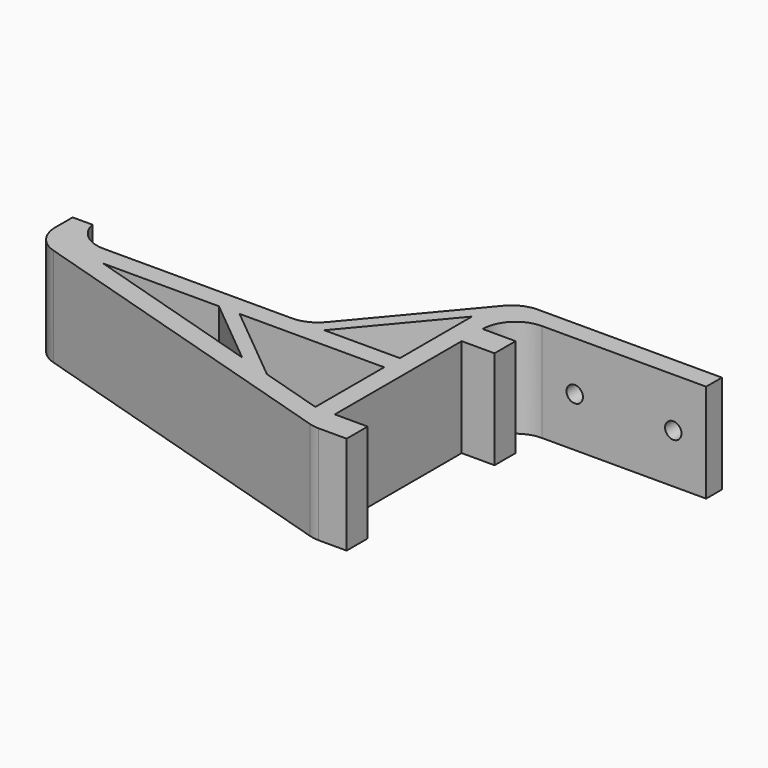
from build123d import *

# Parameters (mm, degrees)
F1_DEPTH    = 15
F2_R        = 1.25
F3_DEPTH    = 40.1383324758
F4_R        = 5
F5_W        = 4
F5_H        = 15
F6_DEPTH    = 5
F8_DEPTH    = 15
F9_T1_DEPTH = 15
F9_T3_DEPTH = 15
F9_T5_DEPTH = 33.4938424429
F9_T7_DEPTH = 18.7397003757


# Not quite as in the source:
# - a fillet or chamfer that OpenCascade refuses, or shapes differently, is made with other operations: its cross-section is extruded or revolved along the edge and cut away or added


with BuildPart() as f1:
    # F0 (on Top) → F1 (new body)
    with BuildSketch(Plane.XY):
        Polygon((0, 20), (0, 23), (-33, 23), (-33, 3), (-83, 3), (-83, 7), (-86, 7), (-86, 0), (-30, -17.1373324758), (-30, -14), (-30, 0), (-30, 20), align=None)
        Polygon((-47.7579661467, -8.5656398223), (-75.7480766687, 0), (-58.1432454597, 0), align=None, mode=Mode.SUBTRACT)
        Polygon((-33, 0), (-33, -13.0819286174), (-42.760486377, -10.0949875429), (-55, 0), align=None, mode=Mode.SUBTRACT)
    extrude(amount=F1_DEPTH)

    # F2 (on face) → F3 (cut, through all)
    with BuildSketch(Plane(origin=(0, 23, 0), x_dir=(-1, 0, 0), z_dir=(0, 1, 0))):
        with Locations((5, 7.5)):
            Circle(F2_R)
        with Locations((20, 7.5)):
            Circle(F2_R)
    extrude(amount=-F3_DEPTH, mode=Mode.SUBTRACT)

    # F4
    f4_edges = [f1.edges().sort_by_distance(p)[0] for p in [
        (-33, 23, 7.5),
        (-30, 20, 7.5),
    ]]
    fillet(f4_edges, radius=F4_R)

    # F5 (on face) → F6 (join)
    with BuildSketch(Plane.YZ.offset(-30)):
        with Locations((-15.1373324758, 7.5)):
            Rectangle(F5_W, F5_H)
        with Locations((13, 7.5)):
            Rectangle(F5_W, F5_H)
    extrude(amount=F6_DEPTH)

    # F7 (on face) → F8 (join, through all)
    with BuildSketch(Plane.XY.offset(15)):
        with BuildLine():
            Line((-31.8302222156, 21.2139380484), (-47.1135309143, 3))
            Line((-47.1135309143, 3), (-44.5027163357, 3))
            Line((-44.5027163357, 3), (-33, 16.7084035176))
            Line((-33, 16.7084035176), (-33, 18))
            ThreePointArc((-33, 18), (-32.6984631039, 19.7101007166), (-31.8302222156, 21.2139380484))
        make_face()
    extrude(amount=-F8_DEPTH)

    # F9: fillet of radius 5 on 4 edges, made by hand

    # F9_s2 → F9_t1 (join)
    with BuildSketch(Plane.XY):
        with BuildLine():
            ThreePointArc((-78.1010205144, 3), (-81.2632981746, 4.1270166538), (-83, 7))
            Line((-83, 7), (-83, 3))
            Line((-83, 3), (-78.1010205144, 3))
        make_face()
    extrude(amount=F9_T1_DEPTH)

    # F9_s4 → F9_t3 (join)
    with BuildSketch(Plane.XY):
        with BuildLine():
            ThreePointArc((-45.6148469895, 4.7860619516), (-47.3319778964, 3.4684610648), (-49.4450692051, 3))
            Line((-49.4450692051, 3), (-47.1135309143, 3))
            Line((-47.1135309143, 3), (-45.6148469895, 4.7860619516))
        make_face()
    extrude(amount=F9_T3_DEPTH)

    # F9_s6 → F9_t5 (cut)
    with BuildSketch(Plane.XY.offset(-9.2469212215)):
        with BuildLine():
            ThreePointArc((-86, 3.6987684886), (-85.0196828505, 0.7251932363), (-82.4631400875, -1.08236329))
            Line((-82.4631400875, -1.08236329), (-86, 0))
            Line((-86, 0), (-86, 3.6987684886))
        make_face()
    extrude(amount=F9_T5_DEPTH, mode=Mode.SUBTRACT)

    # F9_s8 → F9_t7 (cut)
    with BuildSketch(Plane.XY.offset(-1.8698501879)):
        with BuildLine():
            ThreePointArc((-29.2520599249, -17.1373324758), (-29.9917697014, -17.0823127029), (-30.7152000124, -16.9184642544))
            Line((-30.7152000124, -16.9184642544), (-30, -17.1373324758))
            Line((-30, -17.1373324758), (-29.2520599249, -17.1373324758))
        make_face()
    extrude(amount=F9_T7_DEPTH, mode=Mode.SUBTRACT)


solid = f1.part
